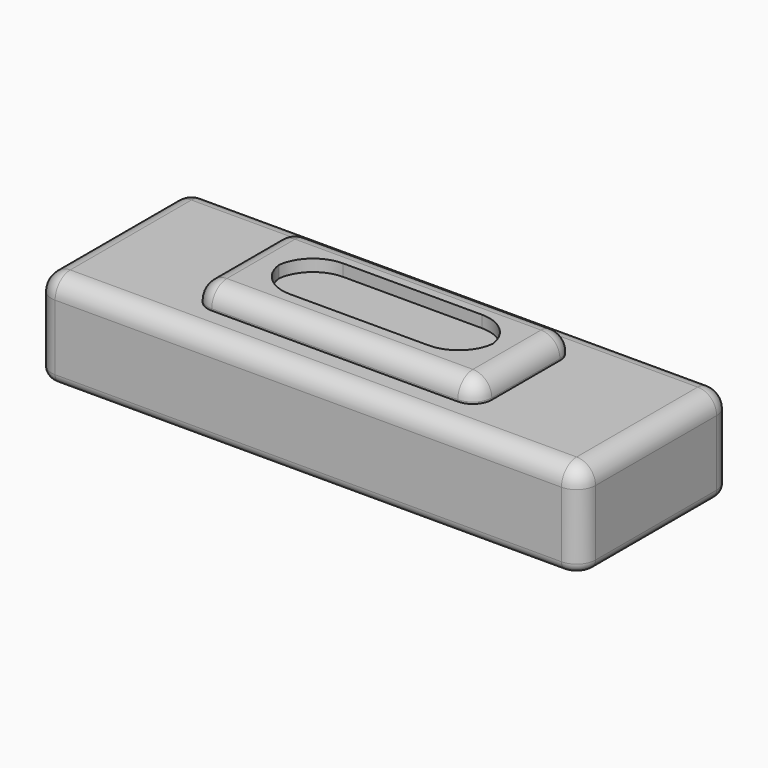
from build123d import *

# Parameters (mm, degrees)
F0_W        = 73.046900332
F0_H        = 12.6124145463
F1_DEPTH    = 12.7
F2_W        = 16.5071599185
F2_H        = 2.7704327367
F3_DEPTH    = 19.05
F4_R        = 2.54
F4_2_R      = 2.54
F5_R        = 2.54
F6_W        = 28.7643400952
F6_H        = 8.9343790896
F7_DEPTH    = 2.54
F8_DEPTH    = 11.938
F9_T1_DEPTH = 2.7704327367
F10_W       = 28.8739772514
F10_H       = 9.0996772051
F11_DEPTH   = 1.27
F12_R       = 2.54
F13_R       = 1.27


# Not quite as in the source:
# - a fillet or chamfer that OpenCascade refuses, or shapes differently, is made with other operations: its cross-section is extruded or revolved along the edge and cut away or added


with BuildPart() as f1:
    # F0 (on Front) → F1 (new body, symmetric)
    with BuildSketch(Plane.XZ):
        Rectangle(F0_W, F0_H)
    extrude(amount=F1_DEPTH, both=True)

    # F4
    f4_edges = [f1.edges().sort_by_distance(p)[0] for p in [
        (-36.52345, 12.7, 0),
        (-36.52345, -12.7, 0),
        (36.52345, 12.7, 0),
        (36.52345, -12.7, 0),
    ]]
    fillet(f4_edges, radius=F4_R)

    # F5
    f5_edges = [f1.edges().sort_by_distance(p)[0] for p in [
        (-35.779501, 11.956051, 6.306207),
    ]]
    fillet(f5_edges, radius=F5_R)

    # F6 (on face) → F7 (cut)
    with BuildSketch(Plane.XY.offset(9.1719310731)):
        with Locations((0.1675928943, 0.0998361502)):
            Rectangle(F6_W, F6_H)
    extrude(amount=F7_DEPTH, mode=Mode.SUBTRACT)

    # F13
    f13_edges = [f1.edges().sort_by_distance(p)[0] for p in [
        (-36.52345, 0, -6.306207),
        (0, -12.7, -6.306207),
        (36.52345, 0, -6.306207),
        (0, 12.7, -6.306207),
        (-35.779501, -11.956051, -6.306207),
        (-35.779501, 11.956051, -6.306207),
        (35.779501, 11.956051, -6.306207),
        (35.779501, -11.956051, -6.306207),
    ]]
    fillet(f13_edges, radius=F13_R)


with BuildPart() as f3:
    # F2 (on Right) → F3 (new body, symmetric)
    with BuildSketch(Plane.YZ):
        with Locations((-0.0095358118, 7.7867147047)):
            Rectangle(F2_W, F2_H)
    extrude(amount=F3_DEPTH, both=True)

    # F4#2
    f4_2_edges = [f3.edges().sort_by_distance(p)[0] for p in [
        (-19.05, -8.263116, 7.786715),
        (19.05, -8.263116, 7.786715),
        (-19.05, 8.244044, 7.786715),
        (19.05, 8.244044, 7.786715),
    ]]
    fillet(f4_2_edges, radius=F4_2_R)

    # F6 (on face) → F8 (cut)
    with BuildSketch(Plane.XY.offset(9.1719310731)):
        with Locations((0.1675928943, 0.0998361502)):
            Rectangle(F6_W, F6_H)
    extrude(amount=-F8_DEPTH, mode=Mode.SUBTRACT)

    # F9: fillet of radius 5.08 on 4 edges, made by hand

    # F9_s2 → F9_t1 (join)
    with BuildSketch(Plane.XY.offset(6.4014983363)):
        with BuildLine():
            ThreePointArc((-9.1345771533, 4.567025695), (-12.7266796018, 3.0791281434), (-14.2145771533, -0.512974305))
            Line((-14.2145771533, -0.512974305), (-14.2145771533, 4.567025695))
            Line((-14.2145771533, 4.567025695), (-9.1345771533, 4.567025695))
        make_face()
        with BuildLine():
            ThreePointArc((14.5497629419, 0.7126466054), (13.0618653903, -2.8794558431), (9.4697629419, -4.3673533946))
            Line((9.4697629419, -4.3673533946), (14.5497629419, -4.3673533946))
            Line((14.5497629419, -4.3673533946), (14.5497629419, 0.7126466054))
        make_face()
        with BuildLine():
            ThreePointArc((-9.1345771533, -4.3673533946), (-12.7266796018, -2.8794558431), (-14.2145771533, 0.7126466054))
            Line((-14.2145771533, 0.7126466054), (-14.2145771533, -4.3673533946))
            Line((-14.2145771533, -4.3673533946), (-9.1345771533, -4.3673533946))
        make_face()
        with BuildLine():
            ThreePointArc((9.4697629419, 4.567025695), (13.0618653903, 3.0791281434), (14.5497629419, -0.512974305))
            Line((14.5497629419, -0.512974305), (14.5497629419, 4.567025695))
            Line((14.5497629419, 4.567025695), (9.4697629419, 4.567025695))
        make_face()
    extrude(amount=F9_T1_DEPTH)

    # F12
    f12_edges = [f3.edges().sort_by_distance(p)[0] for p in [
        (-19.05, -0.009536, 9.171931),
        (-18.306051, -7.519167, 9.171931),
        (-18.306051, 7.500095, 9.171931),
        (0, -8.263116, 9.171931),
        (0, 8.244044, 9.171931),
        (18.306051, -7.519167, 9.171931),
        (18.306051, 7.500095, 9.171931),
        (19.05, -0.009536, 9.171931),
    ]]
    fillet(f12_edges, radius=F12_R)


with BuildPart() as f11:
    # F10 (on face) → F11 (new body)
    with BuildSketch(Plane.XY.offset(6.3062072732)):
        with Locations((0.2010739408, 0.1450735144)):
            Rectangle(F10_W, F10_H)
    extrude(amount=F11_DEPTH)


solid = Compound([f1.part, f3.part, f11.part])
